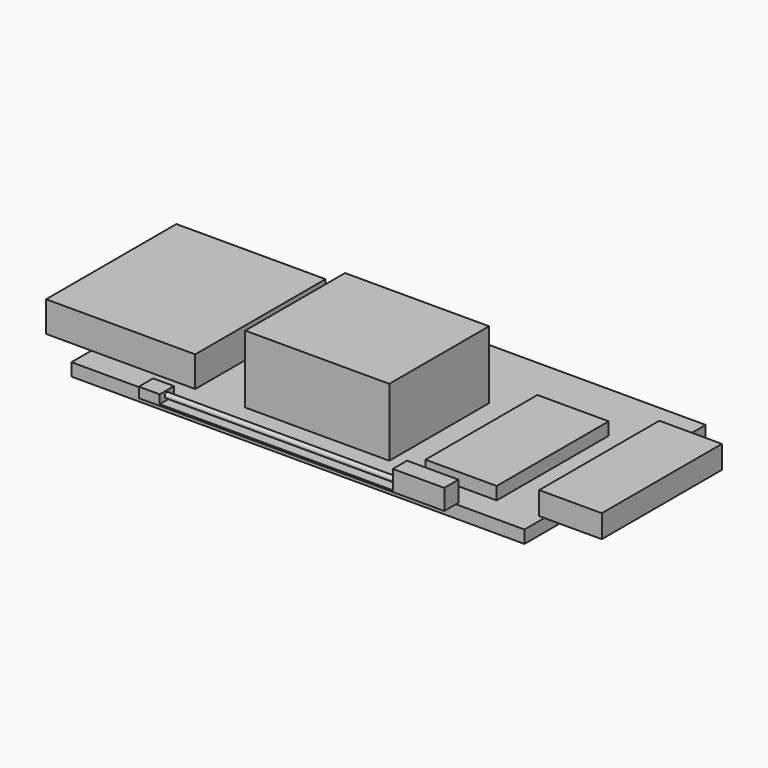
from build123d import *

# Parameters (mm, degrees)
F0_W      = 140
F0_H      = 275
F1_DEPTH  = 25
F0_W_2    = 123
F0_H_2    = 295
F2_DEPTH  = 45
F0_W_3    = 293
F0_H_3    = 320
F3_DEPTH  = 60
F0_W_4    = 283
F0_H_4    = 245
F4_DEPTH  = 133
F5_W      = 890
F5_H      = 445
F6_DEPTH  = 25
F7_W      = 458
F7_H      = 35
F7_W_2    = 41
F7_W_3    = 101
F8_DEPTH  = 3
F9_DEPTH  = 20
F10_DEPTH = 40
F11_R     = 5
F12_DEPTH = 458


with BuildPart() as f1:
    # F0 (on Top) → F1 (new body)
    with BuildSketch(Plane.XY):
        Rectangle(F0_W, F0_H)
    extrude(amount=F1_DEPTH)


with BuildPart() as f2:
    # F0 (on Top) → F2 (new body)
    with BuildSketch(Plane.XY):
        with Locations((214.9233075308, 10)):
            Rectangle(F0_W_2, F0_H_2)
    extrude(amount=F2_DEPTH)


with BuildPart() as f3:
    # F0 (on Top) → F3 (new body)
    with BuildSketch(Plane.XY):
        with Locations((-668.7453899384, 22.5)):
            Rectangle(F0_W_3, F0_H_3)
    extrude(amount=F3_DEPTH)


with BuildPart() as f4:
    # F0 (on Top) → F4 (new body)
    with BuildSketch(Plane.XY):
        with Locations((-282.4815473557, -15)):
            Rectangle(F0_W_4, F0_H_4)
    extrude(amount=F4_DEPTH)


with BuildPart() as f6:
    # F5 (on face) → F6 (new body)
    with BuildSketch(Plane(origin=(0, 0, 0), x_dir=(1, 0, 0), z_dir=(0, 0, -1))):
        with Locations((-281.3649100065, -36.1232197285)):
            Rectangle(F5_W, F5_H)
    extrude(amount=F6_DEPTH)


with BuildPart() as f8:
    # F7 (on Top) → F8 (new body)
    with BuildSketch(Plane.XY):
        with Locations((-300.8197906613, -197.7667400182)):
            Rectangle(F7_W, F7_H)
        with Locations((-550.3197906613, -197.7667400182)):
            Rectangle(F7_W_2, F7_H)
        with Locations((-21.3197906613, -197.7667400182)):
            Rectangle(F7_W_3, F7_H)
    extrude(amount=F8_DEPTH)

    # F7 (on Top) → F9 (join)
    with BuildSketch(Plane.XY):
        with Locations((-550.3197906613, -197.7667400182)):
            Rectangle(F7_W_2, F7_H)
    extrude(amount=F9_DEPTH)

    # F7 (on Top) → F10 (join)
    with BuildSketch(Plane.XY):
        with Locations((-21.3197906613, -197.7667400182)):
            Rectangle(F7_W_3, F7_H)
    extrude(amount=F10_DEPTH)


with BuildPart() as f12:
    # F11 (on face) → F12 (new body, through all)
    with BuildSketch(Plane.YZ.offset(-529.8197906613)):
        with Locations((-197.7667400182, 11.5)):
            Circle(F11_R)
    extrude(amount=F12_DEPTH)


solid = Compound([f1.part, f2.part, f3.part, f4.part, f6.part, f8.part, f12.part])
